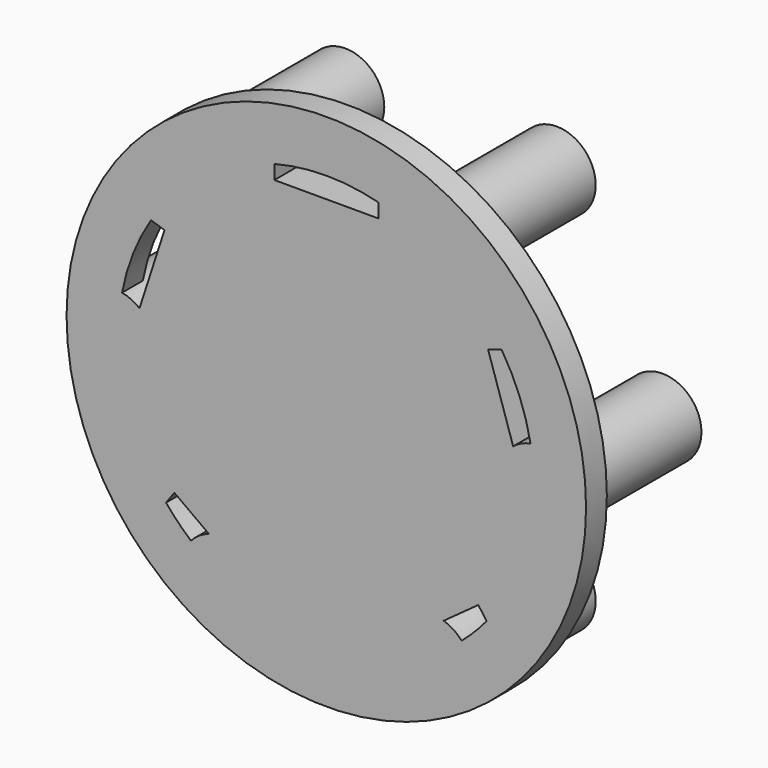
from build123d import *

# Parameters (mm, degrees)
F0_R            = 63.5
F1_DEPTH        = 6.35
F2_DEPTH        = 12.7
F3_R            = 9.5319869965
F4_DEPTH        = 38.1
F4_COPIES_COUNT = 6


# Not quite as in the source:
# - a pattern or mirror of a feature is missing from the dataset's text; its kind, count and spacing are read off the source's solid


with BuildPart() as f1:
    # F0 (on Front) → F1 (new body)
    with BuildSketch(Plane.XZ):
        Circle(F0_R)
        with BuildLine():
            ThreePointArc((50.7040266498, 3.121166689), (50.7760009936, 1.5613209459), (50.8, 0))
            ThreePointArc((50.8, 0), (47.8083719104, -17.1755516731), (39.1858434932, -32.3281559902))
            Line((39.1858434932, -32.3281559902), (40.8804939154, -34.660642193))
            Line((40.8804939154, -34.660642193), (20.3314622583, -49.5903876012))
            Line((20.3314622583, -49.5903876012), (18.636811836, -47.2579013985))
            ThreePointArc((18.636811836, -47.2579013985), (0, -50.8), (-18.636811836, -47.2579013985))
            Line((-18.636811836, -47.2579013985), (-20.3314622583, -49.5903876012))
            Line((-20.3314622583, -49.5903876012), (-40.8804939154, -34.660642193))
            Line((-40.8804939154, -34.660642193), (-39.1858434932, -32.3281559902))
            ThreePointArc((-39.1858434932, -32.3281559902), (-48.3136710278, -15.6980633142), (-50.7040266498, 3.121166689))
            Line((-50.7040266498, 3.121166689), (-53.4460286321, 4.0120971402))
            Line((-53.4460286321, 4.0120971402), (-45.5969969749, 28.1689326541))
            Line((-45.5969969749, 28.1689326541), (-42.8549949926, 27.2780022029))
            ThreePointArc((-42.8549949926, 27.2780022029), (-29.8594908165, 41.0980633142), (-12.7, 49.1868884968))
            Line((-12.7, 49.1868884968), (-12.7, 52.07))
            Line((-12.7, 52.07), (12.7, 52.07))
            Line((12.7, 52.07), (12.7, 49.1868884968))
            ThreePointArc((12.7, 49.1868884968), (29.8594908165, 41.0980633142), (42.8549949926, 27.2780022029))
            Line((42.8549949926, 27.2780022029), (45.5969969749, 28.1689326541))
            Line((45.5969969749, 28.1689326541), (53.4460286321, 4.0120971402))
            Line((53.4460286321, 4.0120971402), (50.7040266498, 3.121166689))
        make_face(mode=Mode.SUBTRACT)
        with BuildLine():
            Line((-20.3314622583, -49.5903876012), (-18.636811836, -47.2579013985))
            ThreePointArc((-18.636811836, -47.2579013985), (-29.8594908165, -41.0980633142), (-39.1858434932, -32.3281559902))
            Line((-39.1858434932, -32.3281559902), (-40.8804939154, -34.660642193))
            Line((-40.8804939154, -34.660642193), (-20.3314622583, -49.5903876012))
        make_face()
        with BuildLine():
            ThreePointArc((-50.7040266498, 3.121166689), (-48.3136710278, 15.6980633142), (-42.8549949926, 27.2780022029))
            Line((-42.8549949926, 27.2780022029), (-45.5969969749, 28.1689326541))
            Line((-45.5969969749, 28.1689326541), (-53.4460286321, 4.0120971402))
            Line((-53.4460286321, 4.0120971402), (-50.7040266498, 3.121166689))
        make_face()
        with BuildLine():
            Line((40.8804939154, -34.660642193), (39.1858434932, -32.3281559902))
            ThreePointArc((39.1858434932, -32.3281559902), (29.8594908165, -41.0980633142), (18.636811836, -47.2579013985))
            Line((18.636811836, -47.2579013985), (20.3314622583, -49.5903876012))
            Line((20.3314622583, -49.5903876012), (40.8804939154, -34.660642193))
        make_face()
        with BuildLine():
            ThreePointArc((42.8549949926, 27.2780022029), (48.3136710278, 15.6980633142), (50.7040266498, 3.121166689))
            Line((50.7040266498, 3.121166689), (53.4460286321, 4.0120971402))
            Line((53.4460286321, 4.0120971402), (45.5969969749, 28.1689326541))
            Line((45.5969969749, 28.1689326541), (42.8549949926, 27.2780022029))
        make_face()
        with BuildLine():
            ThreePointArc((-12.7, 49.1868884968), (0, 50.8), (12.7, 49.1868884968))
            Line((12.7, 49.1868884968), (12.7, 52.07))
            Line((12.7, 52.07), (-12.7, 52.07))
            Line((-12.7, 52.07), (-12.7, 49.1868884968))
        make_face()
    extrude(amount=-F1_DEPTH)

    # F0 (on Front) → F2 (join)
    with BuildSketch(Plane.XZ):
        with BuildLine():
            ThreePointArc((39.1858434932, -32.3281559902), (47.8083719104, -17.1755516731), (50.8, 0))
            ThreePointArc((50.8, 0), (50.7760009936, 1.5613209459), (50.7040266498, 3.121166689))
            Line((50.7040266498, 3.121166689), (47.4068197536, 2.0498392259))
            Line((47.4068197536, 2.0498392259), (39.5577880965, 26.2066747398))
            Line((39.5577880965, 26.2066747398), (42.8549949926, 27.2780022029))
            ThreePointArc((42.8549949926, 27.2780022029), (29.8594908165, 41.0980633142), (12.7, 49.1868884968))
            Line((12.7, 49.1868884968), (12.7, 45.72))
            Line((12.7, 45.72), (-12.7, 45.72))
            Line((-12.7, 45.72), (-12.7, 49.1868884968))
            ThreePointArc((-12.7, 49.1868884968), (-29.8594908165, 41.0980633142), (-42.8549949926, 27.2780022029))
            Line((-42.8549949926, 27.2780022029), (-39.5577880965, 26.2066747398))
            Line((-39.5577880965, 26.2066747398), (-47.4068197536, 2.0498392259))
            Line((-47.4068197536, 2.0498392259), (-50.7040266498, 3.121166689))
            ThreePointArc((-50.7040266498, 3.121166689), (-48.3136710278, -15.6980633142), (-39.1858434932, -32.3281559902))
            Line((-39.1858434932, -32.3281559902), (-37.1480575634, -29.5233842787))
            Line((-37.1480575634, -29.5233842787), (-16.5990259063, -44.4531296869))
            Line((-16.5990259063, -44.4531296869), (-18.636811836, -47.2579013985))
            ThreePointArc((-18.636811836, -47.2579013985), (0, -50.8), (18.636811836, -47.2579013985))
            Line((18.636811836, -47.2579013985), (16.5990259063, -44.4531296869))
            Line((16.5990259063, -44.4531296869), (37.1480575634, -29.5233842787))
            Line((37.1480575634, -29.5233842787), (39.1858434932, -32.3281559902))
        make_face()
    extrude(amount=-F2_DEPTH)

    # F3 (on Front) → F4 (join)
    with BuildSketch(Plane.XZ):
        with Locations((51.6903102398, 0)):
            Circle(F3_R)
    f4 = extrude(amount=-F4_DEPTH)

    # F4_copies: F4 ×6 about axis
    f4_copies_axis = Axis((0, 0, 0), (0, 1, 0))
    for i in range(1, F4_COPIES_COUNT):
        add(f4.rotate(f4_copies_axis, i * 360 / F4_COPIES_COUNT))


solid = f1.part
